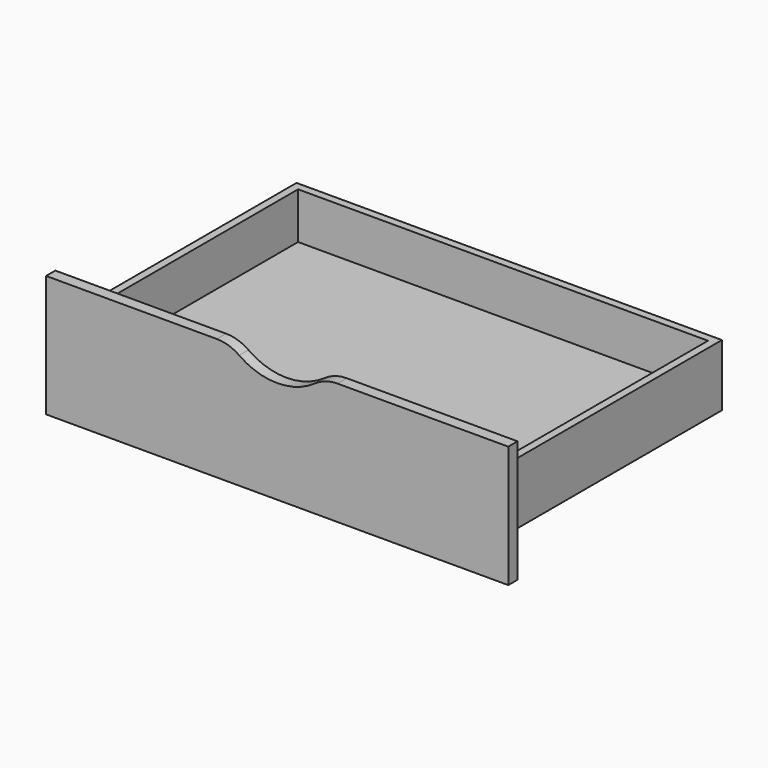
from build123d import *

# Parameters (mm, degrees)
F0_W     = 673.1
F0_H     = 12.7
F1_DEPTH = 101.6
F3_E11_W = 673.1
F3_E11_H = 431.8
F4_DEPTH = 12.7
F5_W     = 698.5
F5_H     = 101.6
F6_DEPTH = 19.05


with BuildPart() as f1:
    # F0 (on Top) → F1 (new body)
    with BuildSketch(Plane.XY):
        Polygon((336.55, 215.9), (349.25, 228.6), (-349.25, 228.6), (-336.55, 215.9), align=None)
        Polygon((349.25, -228.6), (349.25, 228.6), (336.55, 215.9), (336.55, -215.9), (336.55, -228.6), align=None)
        Polygon((-336.55, 215.9), (-349.25, 228.6), (-349.25, -228.6), (-336.55, -228.6), (-336.55, -215.9), align=None)
        with Locations((0, -222.25)):
            Rectangle(F0_W, F0_H)
    extrude(amount=F1_DEPTH)

    # F3_E11 (on explicit) → F4 (join)
    with BuildSketch(Plane(origin=(336.55, 215.9, 12.7), x_dir=(-1, 0, 0), z_dir=(0, 0, 1))):
        with Locations((336.55, 215.9)):
            Rectangle(F3_E11_W, F3_E11_H)
    extrude(amount=F4_DEPTH)

    # F5 (on face) → F6 (join)
    with BuildSketch(Plane.XZ.offset(228.6)):
        with BuildLine():
            Line((-379.476, -49.276), (379.476, -49.276))
            Line((379.476, -49.276), (379.476, 150.876))
            Line((379.476, 150.876), (99.0458770515, 150.876))
            ThreePointArc((99.0458770515, 150.876), (79.7868016321, 147.884991183), (62.3420274532, 139.1937327241))
            ThreePointArc((62.3420274532, 139.1937327241), (0, 119.3512302291), (-62.3420274532, 139.1937327241))
            ThreePointArc((-62.3420274532, 139.1937327241), (-79.7868016321, 147.884991183), (-99.0458770515, 150.876))
            Line((-99.0458770515, 150.876), (-379.476, 150.876))
            Line((-379.476, 150.876), (-379.476, -49.276))
        make_face()
        with Locations((0, 50.8)):
            Rectangle(F5_W, F5_H, mode=Mode.SUBTRACT)
        with Locations((0, 50.8)):
            Rectangle(F5_W, F5_H)
    extrude(amount=F6_DEPTH)


solid = f1.part
